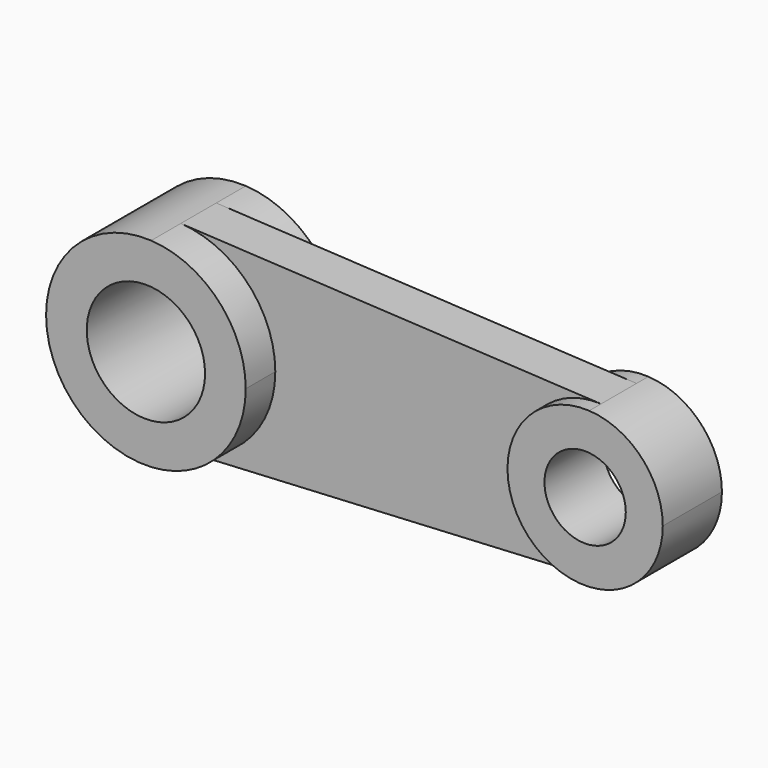
from build123d import *

# Parameters (mm, degrees)
F0_R     = 25.4
F1_DEPTH = 25.4
F2_DEPTH = 9.525
F0_R_2   = 17.4625
F3_DEPTH = 15.875


with BuildPart() as f1:
    # F0 (on Front) → F1 (new body, symmetric)
    with BuildSketch(Plane.XZ):
        with BuildLine():
            ThreePointArc((2.255921, -42.803092), (31.095726, -29.499996), (42.8625, 0))
            ThreePointArc((42.8625, 0), (31.095726, 29.499996), (2.255921, 42.803092))
            ThreePointArc((2.255921, 42.803092), (-42.8625, 0), (2.255921, -42.803092))
        make_face()
        Circle(F0_R, mode=Mode.SUBTRACT)
    extrude(amount=F1_DEPTH, both=True)

    # F0 (on Front) → F2 (join, symmetric)
    with BuildSketch(Plane.XZ):
        with BuildLine():
            ThreePointArc((2.255921, 42.803092), (31.095726, 29.499996), (42.8625, 0))
            ThreePointArc((42.8625, 0), (31.095726, -29.499996), (2.255921, -42.803092))
            Line((2.255921, -42.803092), (182.729605, -33.291294))
            ThreePointArc((182.729605, -33.291294), (147.6375, 0), (182.729605, 33.291294))
            Line((182.729605, 33.291294), (2.255921, 42.803092))
        make_face()
    extrude(amount=F2_DEPTH, both=True)

    # F0 (on Front) → F3 (join, symmetric)
    with BuildSketch(Plane.XZ):
        with BuildLine():
            ThreePointArc((214.3125, 0), (205.160564, 22.944441), (182.729605, 33.291294))
            ThreePointArc((182.729605, 33.291294), (147.6375, 0), (182.729605, -33.291294))
            ThreePointArc((182.729605, -33.291294), (205.160564, -22.944441), (214.3125, 0))
        make_face()
        with Locations((180.975, 0)):
            Circle(F0_R_2, mode=Mode.SUBTRACT)
    extrude(amount=F3_DEPTH, both=True)


solid = f1.part
